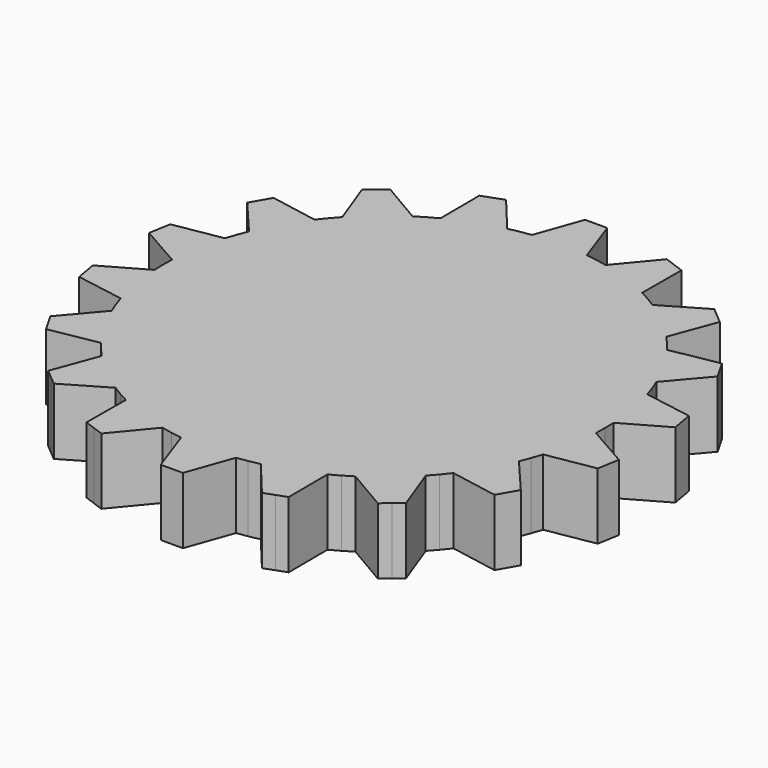
from build123d import *

# Parameters (mm, degrees)
F1_DEPTH = 6


# Not quite as in the source:
# - a feature names something its author has since deleted; it is built from what else it names


with BuildPart() as f1:
    # F0 (on Top) → F1 (new body)
    with BuildSketch(Plane.XY):
        with BuildLine():
            Line((19.975, -0.9996874512), (20, 0))
            Line((20, 0), (19.975, 0.9996874512))
            ThreePointArc((19.975, 0.9996874512), (19.6961550602, 3.4729635533), (19.1122733455, 5.892453442))
            Line((19.1122733455, 5.892453442), (18.7938524157, 6.8404028665))
            Line((18.7938524157, 6.8404028665), (18.4284468549, 7.7712512839))
            ThreePointArc((18.4284468549, 7.7712512839), (17.3205080757, 10), (15.9443244585, 12.0738774867))
            Line((15.9443244585, 12.0738774867), (15.3208888624, 12.8557521937))
            Line((15.3208888624, 12.8557521937), (14.6591510441, 13.6054875203))
            ThreePointArc((14.6591510441, 13.6054875203), (12.8557521937, 15.3208888624), (10.8532547285, 16.799013715))
            Line((10.8532547285, 16.799013715), (10, 17.3205080757))
            Line((10, 17.3205080757), (9.1217452715, 17.7987011662))
            ThreePointArc((9.1217452715, 17.7987011662), (6.8404028665, 18.7938524157), (4.4531223014, 19.4979409623))
            Line((4.4531223014, 19.4979409623), (3.4729635533, 19.6961550602))
            Line((3.4729635533, 19.6961550602), (2.4841223964, 19.8451287705))
            ThreePointArc((2.4841223964, 19.8451287705), (0, 20), (-2.4841223964, 19.8451287705))
            Line((-2.4841223964, 19.8451287705), (-3.4729635533, 19.6961550602))
            Line((-3.4729635533, 19.6961550602), (-4.4531223014, 19.4979409623))
            ThreePointArc((-4.4531223014, 19.4979409623), (-6.8404028665, 18.7938524157), (-9.1217452715, 17.7987011662))
            Line((-9.1217452715, 17.7987011662), (-10, 17.3205080757))
            Line((-10, 17.3205080757), (-10.8532547285, 16.799013715))
            ThreePointArc((-10.8532547285, 16.799013715), (-12.8557521937, 15.3208888624), (-14.6591510441, 13.6054875203))
            Line((-14.6591510441, 13.6054875203), (-15.3208888624, 12.8557521937))
            Line((-15.3208888624, 12.8557521937), (-15.9443244585, 12.0738774867))
            ThreePointArc((-15.9443244585, 12.0738774867), (-17.3205080757, 10), (-18.4284468549, 7.7712512839))
            Line((-18.4284468549, 7.7712512839), (-18.7938524157, 6.8404028665))
            Line((-18.7938524157, 6.8404028665), (-19.1122733455, 5.892453442))
            ThreePointArc((-19.1122733455, 5.892453442), (-19.6961550602, 3.4729635533), (-19.975, 0.9996874512))
            Line((-19.975, 0.9996874512), (-20, 0))
            Line((-20, 0), (-19.975, -0.9996874512))
            ThreePointArc((-19.975, -0.9996874512), (-19.6961550602, -3.4729635533), (-19.1122733455, -5.892453442))
            Line((-19.1122733455, -5.892453442), (-18.7938524157, -6.8404028665))
            Line((-18.7938524157, -6.8404028665), (-18.4284468549, -7.7712512839))
            ThreePointArc((-18.4284468549, -7.7712512839), (-17.3205080757, -10), (-15.9443244585, -12.0738774867))
            Line((-15.9443244585, -12.0738774867), (-15.3208888624, -12.8557521937))
            Line((-15.3208888624, -12.8557521937), (-14.6591510441, -13.6054875203))
            ThreePointArc((-14.6591510441, -13.6054875203), (-12.8557521937, -15.3208888624), (-10.8532547285, -16.799013715))
            Line((-10.8532547285, -16.799013715), (-10, -17.3205080757))
            Line((-10, -17.3205080757), (-9.1217452715, -17.7987011662))
            ThreePointArc((-9.1217452715, -17.7987011662), (-6.8404028665, -18.7938524157), (-4.4531223014, -19.4979409623))
            Line((-4.4531223014, -19.4979409623), (-3.4729635533, -19.6961550602))
            Line((-3.4729635533, -19.6961550602), (-2.4841223964, -19.8451287705))
            ThreePointArc((-2.4841223964, -19.8451287705), (0, -20), (2.4841223964, -19.8451287705))
            Line((2.4841223964, -19.8451287705), (3.4729635533, -19.6961550602))
            Line((3.4729635533, -19.6961550602), (4.4531223014, -19.4979409623))
            ThreePointArc((4.4531223014, -19.4979409623), (6.8404028665, -18.7938524157), (9.1217452715, -17.7987011662))
            Line((9.1217452715, -17.7987011662), (10, -17.3205080757))
            Line((10, -17.3205080757), (10.8532547285, -16.799013715))
            ThreePointArc((10.8532547285, -16.799013715), (12.8557521937, -15.3208888624), (14.6591510441, -13.6054875203))
            Line((14.6591510441, -13.6054875203), (15.3208888624, -12.8557521937))
            Line((15.3208888624, -12.8557521937), (15.9443244585, -12.0738774867))
            ThreePointArc((15.9443244585, -12.0738774867), (17.3205080757, -10), (18.4284468549, -7.7712512839))
            Line((18.4284468549, -7.7712512839), (18.7938524157, -6.8404028665))
            Line((18.7938524157, -6.8404028665), (19.1122733455, -5.892453442))
            ThreePointArc((19.1122733455, -5.892453442), (19.6961550602, -3.4729635533), (19.975, -0.9996874512))
        make_face()
        with BuildLine():
            ThreePointArc((-2.4841223964, 19.8451287705), (0, 20), (2.4841223964, 19.8451287705))
            Line((2.4841223964, 19.8451287705), (1, 24))
            Line((1, 24), (0, 24))
            Line((0, 24), (-1, 24))
            Line((-1, 24), (-2.4841223964, 19.8451287705))
        make_face()
        with BuildLine():
            ThreePointArc((4.4531223014, 19.4979409623), (6.8404028665, 18.7938524157), (9.1217452715, 17.7987011662))
            Line((9.1217452715, 17.7987011662), (9.1481760606, 22.2106027555))
            Line((9.1481760606, 22.2106027555), (8.2084834398, 22.5526228989))
            Line((8.2084834398, 22.5526228989), (7.268790819, 22.8946430422))
            Line((7.268790819, 22.8946430422), (4.4531223014, 19.4979409623))
        make_face()
        with BuildLine():
            ThreePointArc((10.8532547285, 16.799013715), (12.8557521937, 15.3208888624), (14.6591510441, 13.6054875203))
            Line((14.6591510441, 13.6054875203), (16.1929470756, 17.7422790252))
            Line((16.1929470756, 17.7422790252), (15.4269026325, 18.3850666349))
            Line((15.4269026325, 18.3850666349), (14.6608581894, 19.0278542445))
            Line((14.6608581894, 19.0278542445), (10.8532547285, 16.799013715))
        make_face()
        with BuildLine():
            ThreePointArc((15.9443244585, 12.0738774867), (17.3205080757, 10), (18.4284468549, 7.7712512839))
            Line((18.4284468549, 7.7712512839), (21.2846096908, 11.1339745962))
            Line((21.2846096908, 11.1339745962), (20.7846096908, 12))
            Line((20.7846096908, 12), (20.2846096908, 12.8660254038))
            Line((20.2846096908, 12.8660254038), (15.9443244585, 12.0738774867))
        make_face()
        with BuildLine():
            ThreePointArc((19.1122733455, 5.892453442), (19.6961550602, 3.4729635533), (19.975, 0.9996874512))
            Line((19.975, 0.9996874512), (23.80903425, 3.182748511))
            Line((23.80903425, 3.182748511), (23.6353860723, 4.167556264))
            Line((23.6353860723, 4.167556264), (23.4617378946, 5.152364017))
            Line((23.4617378946, 5.152364017), (19.1122733455, 5.892453442))
        make_face()
        with BuildLine():
            Line((23.80903425, -3.182748511), (19.975, -0.9996874512))
            ThreePointArc((19.975, -0.9996874512), (19.6961550602, -3.4729635533), (19.1122733455, -5.892453442))
            Line((19.1122733455, -5.892453442), (23.4617378946, -5.152364017))
            Line((23.4617378946, -5.152364017), (23.6353860723, -4.167556264))
            Line((23.6353860723, -4.167556264), (23.80903425, -3.182748511))
        make_face()
        with BuildLine():
            Line((21.2846096908, -11.1339745962), (18.4284468549, -7.7712512839))
            ThreePointArc((18.4284468549, -7.7712512839), (17.3205080757, -10), (15.9443244585, -12.0738774867))
            Line((15.9443244585, -12.0738774867), (20.2846096908, -12.8660254038))
            Line((20.2846096908, -12.8660254038), (20.7846096908, -12))
            Line((20.7846096908, -12), (21.2846096908, -11.1339745962))
        make_face()
        with BuildLine():
            Line((16.1929470756, -17.7422790252), (14.6591510441, -13.6054875203))
            ThreePointArc((14.6591510441, -13.6054875203), (12.8557521937, -15.3208888624), (10.8532547285, -16.799013715))
            Line((10.8532547285, -16.799013715), (14.6608581894, -19.0278542445))
            Line((14.6608581894, -19.0278542445), (15.4269026325, -18.3850666349))
            Line((15.4269026325, -18.3850666349), (16.1929470756, -17.7422790252))
        make_face()
        with BuildLine():
            Line((9.1481760606, -22.2106027555), (9.1217452715, -17.7987011662))
            ThreePointArc((9.1217452715, -17.7987011662), (6.8404028665, -18.7938524157), (4.4531223014, -19.4979409623))
            Line((4.4531223014, -19.4979409623), (7.268790819, -22.8946430422))
            Line((7.268790819, -22.8946430422), (8.2084834398, -22.5526228989))
            Line((8.2084834398, -22.5526228989), (9.1481760606, -22.2106027555))
        make_face()
        with BuildLine():
            Line((1, -24), (2.4841223964, -19.8451287705))
            ThreePointArc((2.4841223964, -19.8451287705), (0, -20), (-2.4841223964, -19.8451287705))
            Line((-2.4841223964, -19.8451287705), (-1, -24))
            Line((-1, -24), (0, -24))
            Line((0, -24), (1, -24))
        make_face()
        with BuildLine():
            Line((-7.268790819, -22.8946430422), (-4.4531223014, -19.4979409623))
            ThreePointArc((-4.4531223014, -19.4979409623), (-6.8404028665, -18.7938524157), (-9.1217452715, -17.7987011662))
            Line((-9.1217452715, -17.7987011662), (-9.1481760606, -22.2106027555))
            Line((-9.1481760606, -22.2106027555), (-8.2084834398, -22.5526228989))
            Line((-8.2084834398, -22.5526228989), (-7.268790819, -22.8946430422))
        make_face()
        with BuildLine():
            Line((-14.6608581894, -19.0278542445), (-10.8532547285, -16.799013715))
            ThreePointArc((-10.8532547285, -16.799013715), (-12.8557521937, -15.3208888624), (-14.6591510441, -13.6054875203))
            Line((-14.6591510441, -13.6054875203), (-16.1929470756, -17.7422790252))
            Line((-16.1929470756, -17.7422790252), (-15.4269026325, -18.3850666349))
            Line((-15.4269026325, -18.3850666349), (-14.6608581894, -19.0278542445))
        make_face()
        with BuildLine():
            Line((-20.2846096908, -12.8660254038), (-15.9443244585, -12.0738774867))
            ThreePointArc((-15.9443244585, -12.0738774867), (-17.3205080757, -10), (-18.4284468549, -7.7712512839))
            Line((-18.4284468549, -7.7712512839), (-21.2846096908, -11.1339745962))
            Line((-21.2846096908, -11.1339745962), (-20.7846096908, -12))
            Line((-20.7846096908, -12), (-20.2846096908, -12.8660254038))
        make_face()
        with BuildLine():
            Line((-23.4617378946, -5.152364017), (-19.1122733455, -5.892453442))
            ThreePointArc((-19.1122733455, -5.892453442), (-19.6961550602, -3.4729635533), (-19.975, -0.9996874512))
            Line((-19.975, -0.9996874512), (-23.80903425, -3.182748511))
            Line((-23.80903425, -3.182748511), (-23.6353860723, -4.167556264))
            Line((-23.6353860723, -4.167556264), (-23.4617378946, -5.152364017))
        make_face()
        with BuildLine():
            ThreePointArc((-19.975, 0.9996874512), (-19.6961550602, 3.4729635533), (-19.1122733455, 5.892453442))
            Line((-19.1122733455, 5.892453442), (-23.4617378946, 5.152364017))
            Line((-23.4617378946, 5.152364017), (-23.6353860723, 4.167556264))
            Line((-23.6353860723, 4.167556264), (-23.80903425, 3.182748511))
            Line((-23.80903425, 3.182748511), (-19.975, 0.9996874512))
        make_face()
        with BuildLine():
            ThreePointArc((-18.4284468549, 7.7712512839), (-17.3205080757, 10), (-15.9443244585, 12.0738774867))
            Line((-15.9443244585, 12.0738774867), (-20.2846096908, 12.8660254038))
            Line((-20.2846096908, 12.8660254038), (-20.7846096908, 12))
            Line((-20.7846096908, 12), (-21.2846096908, 11.1339745962))
            Line((-21.2846096908, 11.1339745962), (-18.4284468549, 7.7712512839))
        make_face()
        with BuildLine():
            ThreePointArc((-14.6591510441, 13.6054875203), (-12.8557521937, 15.3208888624), (-10.8532547285, 16.799013715))
            Line((-10.8532547285, 16.799013715), (-14.6608581894, 19.0278542445))
            Line((-14.6608581894, 19.0278542445), (-15.4269026325, 18.3850666349))
            Line((-15.4269026325, 18.3850666349), (-16.1929470756, 17.7422790252))
            Line((-16.1929470756, 17.7422790252), (-14.6591510441, 13.6054875203))
        make_face()
        with BuildLine():
            ThreePointArc((-9.1217452715, 17.7987011662), (-6.8404028665, 18.7938524157), (-4.4531223014, 19.4979409623))
            Line((-4.4531223014, 19.4979409623), (-7.268790819, 22.8946430422))
            Line((-7.268790819, 22.8946430422), (-8.2084834398, 22.5526228989))
            Line((-8.2084834398, 22.5526228989), (-9.1481760606, 22.2106027555))
            Line((-9.1481760606, 22.2106027555), (-9.1217452715, 17.7987011662))
        make_face()
    extrude(amount=F1_DEPTH)


solid = f1.part
